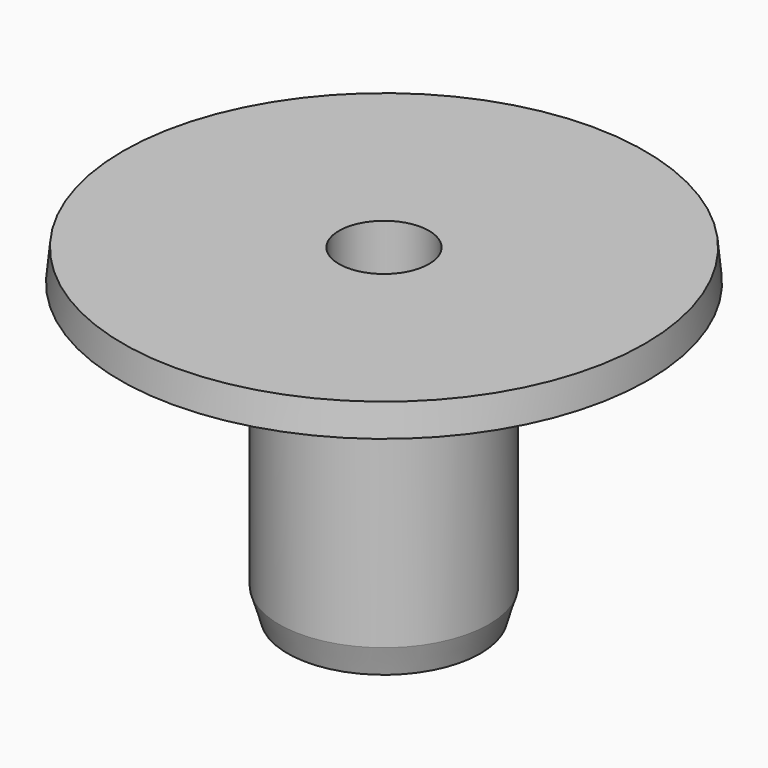
from build123d import *

# Parameters (mm, degrees)
F0_R     = 18.5
F1_DEPTH = 52
F2_SIZE2 = 1.5
F2_SIZE  = 5
F3_R     = 47
F4_DEPTH = 5.5
F6_R     = 7.9375
F7_DEPTH = 57.501


# Not quite as in the source:
# - a fillet or chamfer that OpenCascade refuses, or shapes differently, is made with other operations: its cross-section is extruded or revolved along the edge and cut away or added


with BuildPart() as f1:
    # F0 (on Top) → F1 (new body)
    with BuildSketch(Plane.XY):
        Circle(F0_R)
    extrude(amount=F1_DEPTH)

    # F2
    f2_edges = [f1.edges().sort_by_distance(p)[0] for p in [
        (-18.5, 0, 0),
    ]]
    f2_side = f1.faces().sort_by_distance((-18.5, 0, 26))[0]
    chamfer(f2_edges, length=F2_SIZE, length2=F2_SIZE2, reference=f2_side)

    # F3 (on face) → F4 (join)
    with BuildSketch(Plane.XY.offset(52)):
        Circle(F3_R)
    extrude(amount=F4_DEPTH)

    # F5: chamfer of 1 x 10.2 on 1 edges, made by hand

    # F5_s1 → F5_t2 (revolve, cut)
    with BuildSketch(Plane.XZ):
        Polygon((47, 47.3), (46, 57.5), (47, 57.5), align=None)
    revolve(axis=Axis((0, 0, 57.5), (0, 0, 1)), mode=Mode.SUBTRACT)

    # F6 (on face) → F7 (cut, through all)
    with BuildSketch(Plane.XY.offset(57.5)):
        Circle(F6_R)
    extrude(amount=-F7_DEPTH, mode=Mode.SUBTRACT)


solid = f1.part
